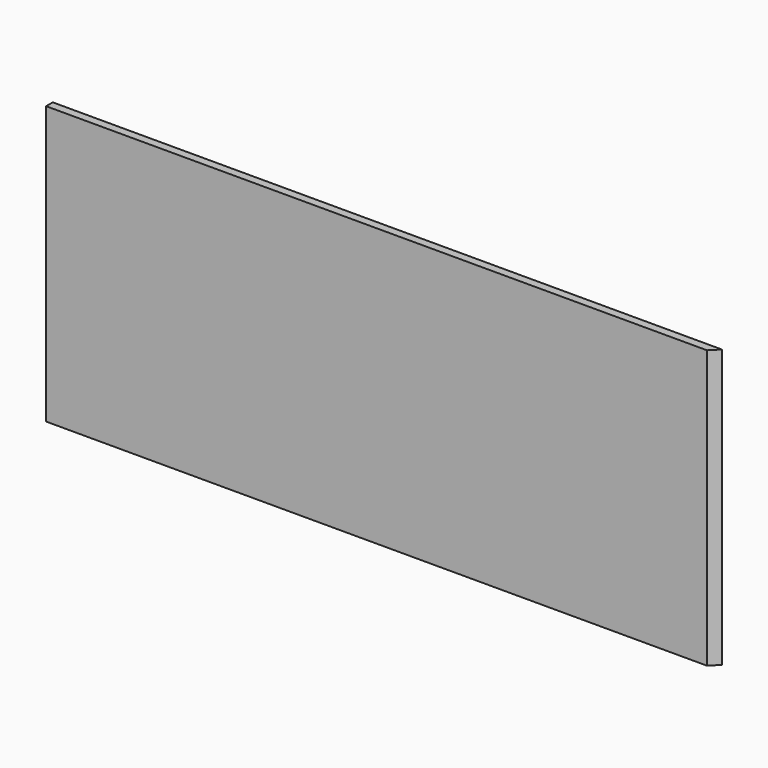
from build123d import *

# Parameters (mm, degrees)
F0_W     = 482
F0_H     = 200
F1_DEPTH = 6
F2_SIZE  = 5.99999


# Not quite as in the source:
# - a fillet or chamfer is up to 0.001 mm smaller than in the source, because OpenCascade refuses the exact size


with BuildPart() as f1:
    # F0 (on Front) → F1 (new body)
    with BuildSketch(Plane.XZ):
        Rectangle(F0_W, F0_H)
    extrude(amount=F1_DEPTH)

    # F2 (size 6 in the source; OpenCascade refuses exactly that, so slightly less here)
    f2_edges = [f1.edges().sort_by_distance(p)[0] for p in [
        (241, -6, 0),
    ]]
    chamfer(f2_edges, length=F2_SIZE)


solid = f1.part
